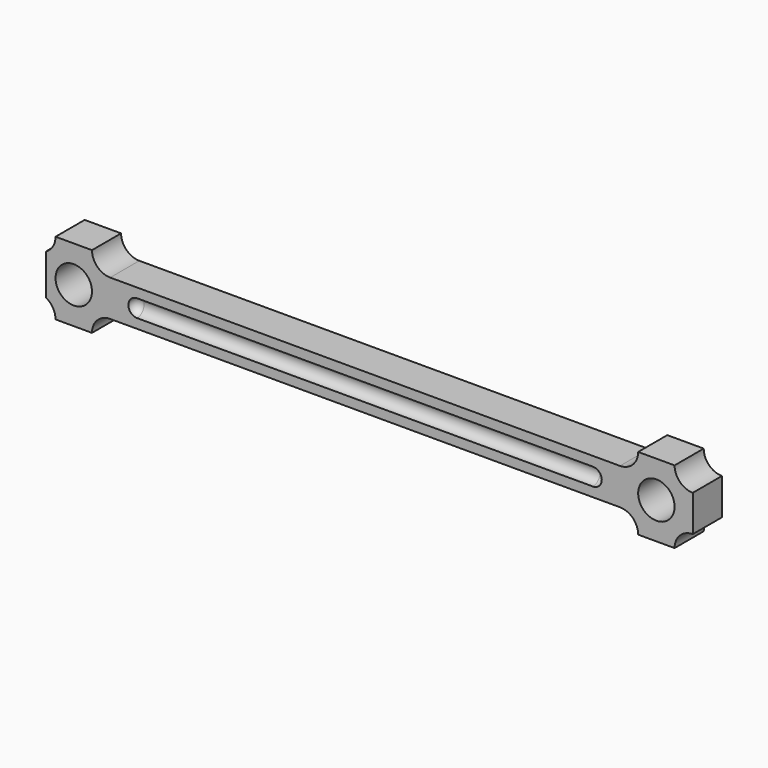
from build123d import *

# Parameters (mm, degrees)
F0_R     = 3.175
F1_DEPTH = 3.175
F3_DEPTH = 41.275
F4_R     = 1.52399


# Not quite as in the source:
# - a fillet or chamfer is up to 0.001 mm smaller than in the source, because OpenCascade refuses the exact size


with BuildPart() as f1:
    # F0 (on Front) → F1 (new body, symmetric)
    with BuildSketch(Plane.XZ):
        with BuildLine():
            Line((44.45, 3.175), (-44.45, 3.175))
            ThreePointArc((-44.45, 3.175), (-46.6950640303, 4.1049359697), (-47.625, 6.35))
            Line((-47.625, 6.35), (-53.975, 6.35))
            ThreePointArc((-53.975, 6.35), (-54.4187617277, 4.7310613044), (-55.626, 3.5646725507))
            Line((-55.626, 3.5646725507), (-55.626, -3.5646725507))
            ThreePointArc((-55.626, -3.5646725507), (-54.4187617277, -4.7310613044), (-53.975, -6.35))
            Line((-53.975, -6.35), (-47.625, -6.35))
            ThreePointArc((-47.625, -6.35), (-46.6950640303, -4.1049359697), (-44.45, -3.175))
            Line((-44.45, -3.175), (44.45, -3.175))
            ThreePointArc((44.45, -3.175), (46.6950640303, -4.1049359697), (47.625, -6.35))
            Line((47.625, -6.35), (53.975, -6.35))
            ThreePointArc((53.975, -6.35), (54.9049359697, -4.1049359697), (57.15, -3.175))
            Line((57.15, -3.175), (57.15, 3.175))
            ThreePointArc((57.15, 3.175), (54.9049359697, 4.1049359697), (53.975, 6.35))
            Line((53.975, 6.35), (47.625, 6.35))
            ThreePointArc((47.625, 6.35), (46.6950640303, 4.1049359697), (44.45, 3.175))
        make_face()
        with Locations((-50.8, 0)):
            Circle(F0_R, mode=Mode.SUBTRACT)
        with Locations((50.8, 0)):
            Circle(F0_R, mode=Mode.SUBTRACT)
    extrude(amount=F1_DEPTH, both=True)

    # F2 (on Right) → F3 (cut, symmetric)
    with BuildSketch(Plane.YZ):
        with BuildLine():
            Line((3.175, -1.524), (3.175, 1.524))
            ThreePointArc((3.175, 1.524), (1.651, 0), (3.175, -1.524))
        make_face()
        with BuildLine():
            Line((-3.175, 1.524), (-3.175, -1.524))
            ThreePointArc((-3.175, -1.524), (-1.651, 0), (-3.175, 1.524))
        make_face()
    extrude(amount=F3_DEPTH, both=True, mode=Mode.SUBTRACT)

    # F4 (radius 1.524 in the source; OpenCascade refuses exactly that, so slightly less here)
    f4_edges = [f1.edges().sort_by_distance(p)[0] for p in [
        (41.275, 1.651, 0),
        (-41.275, 1.651, 0),
        (-41.275, -1.651, 0),
        (41.275, -1.651, 0),
    ]]
    fillet(f4_edges, radius=F4_R)


solid = f1.part
